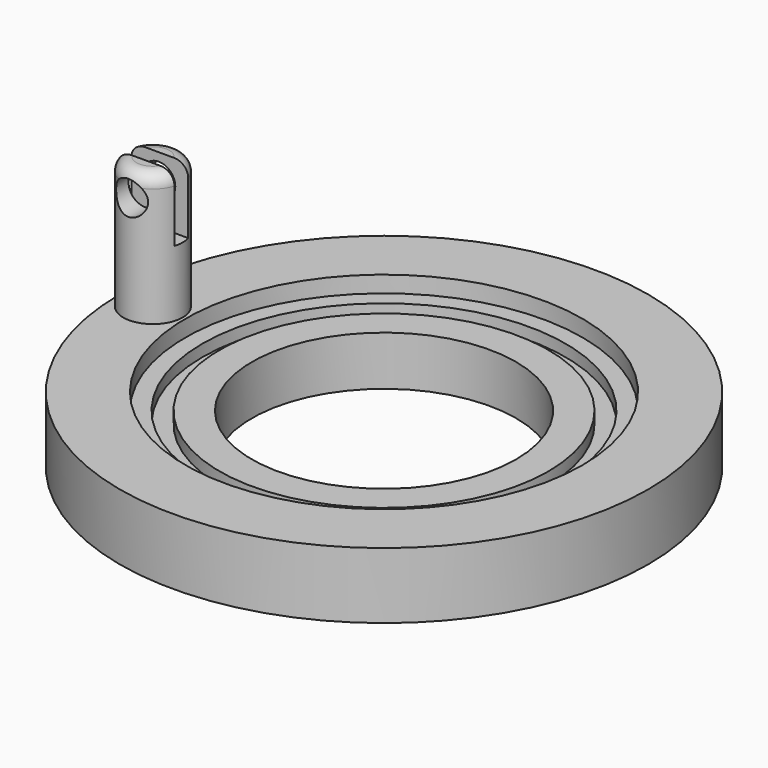
from build123d import *

# Parameters (mm, degrees)
F0_R           = 50.8
F1_DEPTH       = 12.7
F2_R           = 38.1635
F3_DEPTH       = 3.175
F4_R           = 34.925
F4_R_2         = 31.623
F5_DEPTH       = 2.286
F4_R_3         = 25.4
F6_DEPTH       = 9.526
F8_R           = 5.715
F9_DEPTH       = 25.4
F10_R          = 3.175
F11_DEPTH      = 50.801
F11_DEPTH_BACK = 25.4
F13_W          = 3.302
F13_H          = 15.8052066865
F14_DEPTH      = 50.801


# Not quite as in the source:
# - a fillet or chamfer that OpenCascade refuses, or shapes differently, is made with other operations: its cross-section is extruded or revolved along the edge and cut away or added


with BuildPart() as f1:
    # F0 (on Top) → F1 (new body)
    with BuildSketch(Plane.XY):
        Circle(F0_R)
    extrude(amount=F1_DEPTH)

    # F2 (on face) → F3 (cut)
    with BuildSketch(Plane.XY.offset(12.7)):
        Circle(F2_R)
    extrude(amount=-F3_DEPTH, mode=Mode.SUBTRACT)

    # F4 (on face) → F5 (cut)
    with BuildSketch(Plane.XY.offset(9.525)):
        Circle(F4_R)
        Circle(F4_R_2, mode=Mode.SUBTRACT)
    extrude(amount=-F5_DEPTH, mode=Mode.SUBTRACT)

    # F4 (on face) → F6 (cut, through all)
    with BuildSketch(Plane.XY.offset(9.525)):
        Circle(F4_R_3)
    extrude(amount=-F6_DEPTH, mode=Mode.SUBTRACT)

    # F8 (on offset) → F9 (join)
    with BuildSketch(Plane.XY.offset(12.7)):
        with Locations((-44.45, 0)):
            Circle(F8_R)
    extrude(amount=F9_DEPTH)

    # F10 (on Front) → F11 (cut, two sides)
    with BuildSketch(Plane.XZ) as f11_sk:
        with Locations((-44.6398891509, 33.3248)):
            Circle(F10_R)
    extrude(amount=F11_DEPTH, mode=Mode.SUBTRACT)
    extrude(f11_sk.sketch, amount=-F11_DEPTH_BACK, mode=Mode.SUBTRACT)

    # F12: fillet of radius 2.54 on 1 edges, made by hand

    # F12_s1 → F12_t2 (revolve, cut)
    with BuildSketch(Plane.XZ):
        with BuildLine():
            ThreePointArc((-38.735, 35.56), (-39.4789487758, 37.3560512242), (-41.275, 38.1))
            Line((-41.275, 38.1), (-38.735, 38.1))
            Line((-38.735, 38.1), (-38.735, 35.56))
        make_face()
    revolve(axis=Axis((-44.45, 0, 38.1), (0, 0, 1)), mode=Mode.SUBTRACT)

    # F13 (on Right) → F14 (cut, through all)
    with BuildSketch(Plane.YZ):
        with Locations((0, 33.3026033432)):
            Rectangle(F13_W, F13_H)
    extrude(amount=-F14_DEPTH, mode=Mode.SUBTRACT)


solid = f1.part
